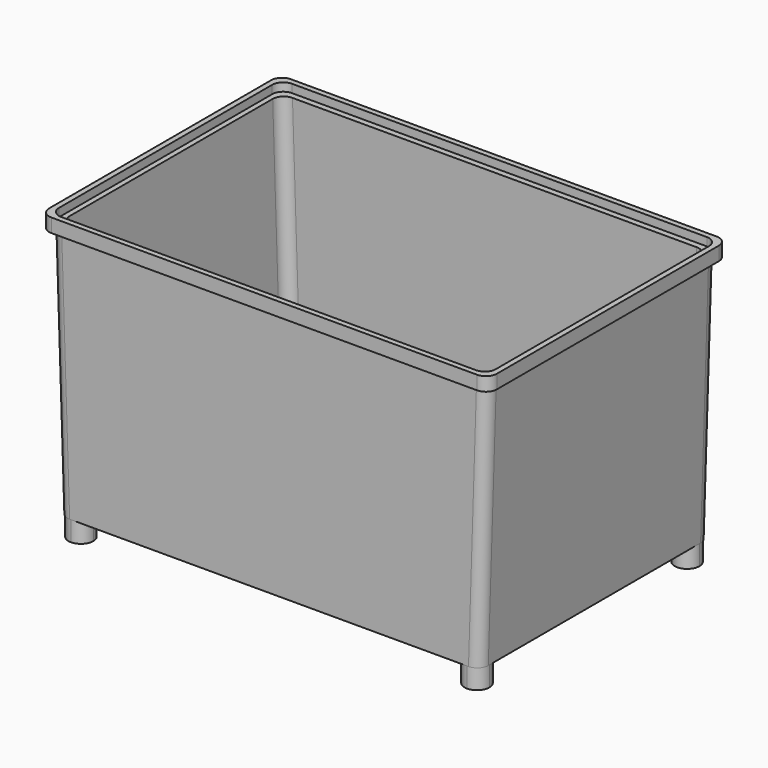
from build123d import *

# Parameters (mm, degrees)
F1_DEPTH = 27.25
F2_DEPTH = 26.15
F4_T     = -1
F5_DEPTH = 3.62
F6_R     = 2


with BuildPart() as f1:
    # F0 (on Front) → F1 (new body, symmetric)
    with BuildSketch(Plane.XZ):
        Polygon((40.75, 10.1086891984), (0, 10.1086891984), (-40.75, 10.1086891984), (-40.75, 7.6086891984), (-39.75, 7.6086891984), (39.75, 7.6086891984), (40.75, 7.6086891984), align=None)
    extrude(amount=F1_DEPTH, both=True)

    # F0 (on Front) → F2 (join, symmetric)
    with BuildSketch(Plane.XZ):
        Polygon((39.75, 7.6086891984), (-39.75, 7.6086891984), (-38.3, -37.8913108016), (0, -37.8913108016), (38.3, -37.8913108016), align=None)
    extrude(amount=F2_DEPTH, both=True)

    # F4
    f4_openings = [f1.faces().sort_by_distance(p)[0] for p in [
        (0, 0, 10.108689),
    ]]
    offset(amount=F4_T, openings=f4_openings, kind=Kind.INTERSECTION)

    # F3 (on face) → F5 (join)
    with BuildSketch(Plane(origin=(0, 0, -37.8913108016), x_dir=(1, 0, 0), z_dir=(0, 0, -1))):
        with BuildLine():
            ThreePointArc((-38.3, 23.9), (-36.05, 21.65), (-33.8, 23.9))
            ThreePointArc((-33.8, 23.9), (-34.4590097351, 25.4909902504), (-36.0499999795, 26.15))
            ThreePointArc((-36.0499999795, 26.15), (-37.6409902504, 25.4909902649), (-38.3, 23.9))
        make_face()
        with BuildLine():
            ThreePointArc((-33.8, -23.9), (-36.0499999898, -21.65), (-38.3, -23.8999999795))
            ThreePointArc((-38.3, -23.8999999795), (-37.6409902649, -25.4909902504), (-36.05, -26.15))
            ThreePointArc((-36.05, -26.15), (-34.4590097423, -25.4909902577), (-33.8, -23.9))
        make_face()
        with BuildLine():
            ThreePointArc((36.05, -26.15), (37.6409902577, -25.4909902577), (38.3, -23.9))
            ThreePointArc((38.3, -23.9), (34.4590097423, -22.3090097423), (36.05, -26.15))
        make_face()
        with BuildLine():
            ThreePointArc((38.3, 23.9), (37.6409902577, 25.4909902577), (36.05, 26.15))
            ThreePointArc((36.05, 26.15), (34.4590097423, 22.3090097423), (38.3, 23.9))
        make_face()
    extrude(amount=F5_DEPTH)

    # F6
    f6_edges = [f1.edges().sort_by_distance(p)[0] for p in [
        (-39.025, -26.15, -15.141311),
        (39.025, -26.15, -15.141311),
        (39.025, 26.15, -15.141311),
        (-39.025, 26.15, -15.141311),
        (-40.75, 27.25, 8.858689),
        (-40.75, -27.25, 8.858689),
        (40.75, -27.25, 8.858689),
        (40.75, 27.25, 8.858689),
        (38.05636, -25.15, -14.141311),
        (-38.05636, -25.15, -14.141311),
        (-38.05636, 25.15, -14.141311),
        (38.05636, 25.15, -14.141311),
        (39.75, 26.25, 9.358689),
        (-39.75, 26.25, 9.358689),
        (39.75, -26.25, 9.358689),
        (-39.75, -26.25, 9.358689),
    ]]
    fillet(f6_edges, radius=F6_R)


solid = f1.part
